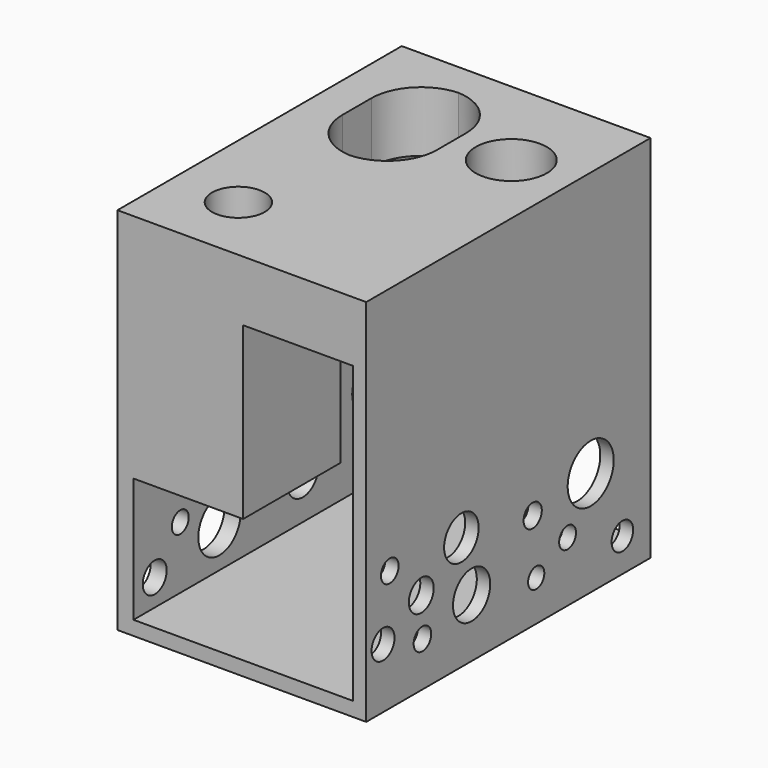
from build123d import *

# Parameters (mm, degrees)
F0_W         = 88.9
F0_H         = 127
F1_DEPTH     = 88.9
F3_DEPTH     = 5.08
F4_DEPTH     = 25.4
F2_W         = 78.3582460135
F2_H         = 44.45
F5_DEPTH     = 120.65
F6_DEPTH     = 25.4
F7_R         = 9.4165633134
F8_DEPTH     = 38.1
F9_DEPTH     = 38.1
F10_DEPTH    = 25.4
F11_DEPTH    = 101.6
F12_R        = 3.7821151403
F13_DEPTH    = 25.4
F14_R        = 8.3394092173
F15_DEPTH    = 25.4
F16_R        = 6.9968499513
F17_DEPTH    = 25.4
F18_R        = 3.8523221967
F19_DEPTH    = 25.4
F20_R        = 9.4524039115
F21_DEPTH    = 25.4
F22_R        = 3.8935430456
F22_R_2      = 2.5048426579
F22_R_3      = 5.3475780775
F22_R_4      = 3.5866360784
F22_R_5      = 3.0785479475
F23_DEPTH    = 25.4
F24_R        = 10.2887517637
F24_R_2      = 3.7572197848
F24_R_3      = 4.8207100709
F24_R_4      = 7.7084596518
F24_R_5      = 4.0689133859
F24_R_6      = 8.3104077663
F24_R_7      = 5.128893449
F24_R_8      = 5.5582930393
F24_R_9      = 3.9454288103
F24_R_10     = 3.6254323416
F24_R_11     = 3.933516476
F25_DEPTH    = 25.4
F27_DEPTH    = 60.96
F28_W        = 33.8233187795
F28_H        = 48.4882295132
F29_DEPTH    = 25.4
F30_T1_DEPTH = 21.59
F31_R        = 12.7015512299
F32_DEPTH    = 25.4


# Not quite as in the source:
# - a fillet or chamfer that OpenCascade refuses, or shapes differently, is made with other operations: its cross-section is extruded or revolved along the edge and cut away or added


with BuildPart() as f1:
    # F0 (on Top) → F1 (new body)
    with BuildSketch(Plane.XY):
        with Locations((44.45, 63.5)):
            Rectangle(F0_W, F0_H)
    extrude(amount=F1_DEPTH)

    # F3 (add): a face of the model
    f3_faces = [f1.faces().sort_by_distance(p)[0] for p in [
        (44.45, 63.5, 0),
    ]]
    extrude(f3_faces, amount=F3_DEPTH)

    # F4 (add): a face of the model
    f4_faces = [f1.faces().sort_by_distance(p)[0] for p in [
        (44.45, 127, 41.91),
    ]]
    extrude(f4_faces, amount=F4_DEPTH)

    # F2 (on face) → F5 (cut)
    with BuildSketch(Plane.XZ):
        with Locations((44.9183965102, 22.225)):
            Rectangle(F2_W, F2_H)
    extrude(amount=-F5_DEPTH, mode=Mode.SUBTRACT)

    # F6 (cut): a face of the model
    f6_faces = [f1.faces().sort_by_distance(p)[0] for p in [
        (44.45, 152.4, 41.91),
    ]]
    extrude(f6_faces, amount=-F6_DEPTH, mode=Mode.SUBTRACT)

    # F7 (on face) → F8 (cut)
    with BuildSketch(Plane.XY.offset(88.9)):
        with Locations((23.3609545976, 24.8096976429)):
            Circle(F7_R)
    extrude(amount=-F8_DEPTH, mode=Mode.SUBTRACT)

    # F9 (add): a face of the model
    f9_faces = [f1.faces().sort_by_distance(p)[0] for p in [
        (44.9835020735, 64.4787714966, 88.9),
    ]]
    extrude(f9_faces, amount=F9_DEPTH)

    # F10 (add): a face of the model
    f10_faces = [f1.faces().sort_by_distance(p)[0] for p in [
        (44.9183965102, 120.65, 22.225),
    ]]
    extrude(f10_faces, amount=F10_DEPTH)

    # F11 (cut): a face of the model
    f11_faces = [f1.faces().sort_by_distance(p)[0] for p in [
        (44.9183965102, 95.25, 22.225),
    ]]
    extrude(f11_faces, amount=-F11_DEPTH, mode=Mode.SUBTRACT)

    # F12 (on face) → F13 (cut)
    with BuildSketch(Plane(origin=(0, 0, 0), x_dir=(0, -1, 0), z_dir=(-1, 0, 0))):
        with Locations((-20.8959858865, 22.2413502634)):
            Circle(F12_R)
    extrude(amount=-F13_DEPTH, mode=Mode.SUBTRACT)

    # F14 (on face) → F15 (cut)
    with BuildSketch(Plane(origin=(0, 0, 0), x_dir=(0, -1, 0), z_dir=(-1, 0, 0))):
        with Locations((-106.0243174434, 31.2219746411)):
            Circle(F14_R)
    extrude(amount=-F15_DEPTH, mode=Mode.SUBTRACT)

    # F16 (on face) → F17 (cut)
    with BuildSketch(Plane(origin=(0, 0, 0), x_dir=(0, -1, 0), z_dir=(-1, 0, 0))):
        with Locations((-75.6411701441, 14.8054044694)):
            Circle(F16_R)
    extrude(amount=-F17_DEPTH, mode=Mode.SUBTRACT)

    # F18 (on face) → F19 (cut)
    with BuildSketch(Plane(origin=(0, 0, 0), x_dir=(0, -1, 0), z_dir=(-1, 0, 0))):
        with Locations((-59.9940270185, 33.8436961174)):
            Circle(F18_R)
    extrude(amount=-F19_DEPTH, mode=Mode.SUBTRACT)

    # F20 (on face) → F21 (cut)
    with BuildSketch(Plane.YZ.offset(5.7392735034)):
        with Locations((38.390211761, 14.1541231424)):
            Circle(F20_R)
    extrude(amount=-F21_DEPTH, mode=Mode.SUBTRACT)

    # F22 (on face) → F23 (cut)
    with BuildSketch(Plane.YZ.offset(5.7392735034)):
        with Locations((103.7926003337, 9.5047177747)):
            Circle(F22_R)
        with Locations((29.4643323869, 32.8702926636)):
            Circle(F22_R_2)
        with Locations((9.4724670053, 9.5047177747)):
            Circle(F22_R_3)
        with Locations((47.9597039521, 26.7663411796)):
            Circle(F22_R_4)
        with Locations((75.3153562546, 34.4844758511)):
            Circle(F22_R_5)
    extrude(amount=-F23_DEPTH, mode=Mode.SUBTRACT)

    # F24 (on face) → F25 (cut)
    with BuildSketch(Plane(origin=(84.0975195169, 0, 0), x_dir=(0, -1, 0), z_dir=(-1, 0, 0))):
        with Locations((-100.267700851, 32.3584228754)):
            Circle(F24_R)
        with Locations((-89.9443402886, 16.390549019)):
            Circle(F24_R_2)
        with Locations((-114.4196018577, 6.8739750423)):
            Circle(F24_R_3)
        with Locations((-42.5033308566, 35.6052704155)):
            Circle(F24_R_4)
        with Locations((-74.3665918708, 29.6205114573)):
            Circle(F24_R_5)
        with Locations((-47.0789894462, 15.7656241208)):
            Circle(F24_R_6)
        with Locations((-7.5106075965, 16.2924602628)):
            Circle(F24_R_7)
        with Locations((-24.5902761817, 24.7659608722)):
            Circle(F24_R_8)
        with Locations((-10.5220889673, 38.1775014102)):
            Circle(F24_R_9)
        with Locations((-75.9231299162, 9.4177098945)):
            Circle(F24_R_10)
        with Locations((-25.1116491854, 10.8577311039)):
            Circle(F24_R_11)
    extrude(amount=-F25_DEPTH, mode=Mode.SUBTRACT)

    # F26 (on face) → F27 (cut)
    with BuildSketch(Plane(origin=(0, 0, 44.45), x_dir=(1, 0, 0), z_dir=(0, 0, -1))):
        Polygon((84.0975195169, 0), (44.9183965102, 0), (44.9183965102, -43.4251762927), (5.7392735034, -43.4251762927), (5.7392735034, -127), (84.0975195169, -127), align=None)
    extrude(amount=-F27_DEPTH, mode=Mode.SUBTRACT)

    # F28 (on face) → F29 (cut)
    with BuildSketch(Plane.XY.offset(127)):
        with Locations((29.9662053585, 90.6256511807)):
            Rectangle(F28_W, F28_H)
    extrude(amount=-F29_DEPTH, mode=Mode.SUBTRACT)

    # F30: fillet of radius 17.78 on 4 edges, made by hand

    # F30_s2 → F30_t1 (join)
    with BuildSketch(Plane.XY.offset(105.41)):
        with BuildLine():
            ThreePointArc((29.0978647482, 66.3815364242), (41.6702233177, 71.5891778547), (46.8778647482, 84.1615364242))
            Line((46.8778647482, 84.1615364242), (46.8778647482, 66.3815364242))
            Line((46.8778647482, 66.3815364242), (29.0978647482, 66.3815364242))
        make_face()
        with BuildLine():
            ThreePointArc((13.0545459688, 84.1615364242), (18.2621873993, 71.5891778547), (30.8345459688, 66.3815364242))
            Line((30.8345459688, 66.3815364242), (13.0545459688, 66.3815364242))
            Line((13.0545459688, 66.3815364242), (13.0545459688, 84.1615364242))
        make_face()
        with BuildLine():
            ThreePointArc((29.0978647482, 114.8697659373), (41.6702233177, 109.6621245068), (46.8778647482, 97.0897659373))
            Line((46.8778647482, 97.0897659373), (46.8778647482, 114.8697659373))
            Line((46.8778647482, 114.8697659373), (29.0978647482, 114.8697659373))
        make_face()
        with BuildLine():
            ThreePointArc((30.8345459688, 114.8697659373), (18.2621873993, 109.6621245068), (13.0545459688, 97.0897659373))
            Line((13.0545459688, 97.0897659373), (13.0545459688, 114.8697659373))
            Line((13.0545459688, 114.8697659373), (30.8345459688, 114.8697659373))
        make_face()
    extrude(amount=F30_T1_DEPTH)

    # F31 (on face) → F32 (cut)
    with BuildSketch(Plane.XY.offset(127)):
        with Locations((66.893927753, 92.3067107797)):
            Circle(F31_R)
    extrude(amount=-F32_DEPTH, mode=Mode.SUBTRACT)


solid = f1.part
